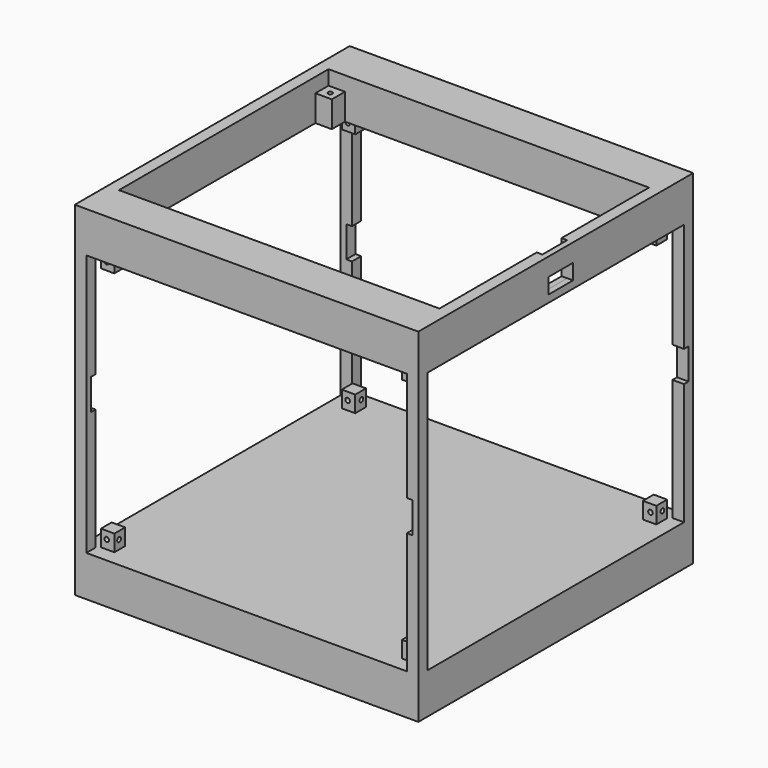
from build123d import *

# Parameters (mm, degrees)
F0_W      = 114.3
F0_H      = 114.3
F1_DEPTH  = 114.3
F2_W      = 5.08
F2_H      = 5.08
F2_R      = 0.762
F2_W_2    = 0.396875
F2_H_2    = 76.2
F3_DEPTH  = 4.826
F2_W_3    = 95.6818
F2_H_3    = 0.396875
F2_H_4    = 30.908625
F2_H_5    = 9.525
F2_H_6    = 34.972625
F4_DEPTH  = 25.4
F2_W_4    = 1.482725
F6_DEPTH  = 11.166475
F5_W      = 10.31875
F5_H      = 5.16255
F7_DEPTH  = 25.4
F11_W     = 5.08
F11_H     = 5.08
F11_R     = 0.762
F12_DEPTH = 4.826
F11_W_2   = 95.6818
F11_H_2   = 0.396875
F11_W_3   = 0.396875
F11_H_3   = 30.908625
F11_H_4   = 34.972625
F11_H_5   = 9.525
F11_H_6   = 76.2
F13_DEPTH = 76.2
F10_W     = 5.08
F10_H     = 5.08
F10_R     = 0.762
F14_DEPTH = 4.826
F10_W_2   = 95.6818
F10_H_2   = 0.396875
F10_W_3   = 0.396875
F10_H_3   = 76.2
F10_H_4   = 34.972625
F10_H_5   = 9.525
F10_H_6   = 30.908625
F15_DEPTH = 50.8
F9_W      = 5.08
F9_H      = 5.08
F9_R      = 0.762
F16_DEPTH = 4.826
F9_W_2    = 95.6818
F9_H_2    = 0.396875
F9_W_3    = 0.396875
F9_H_3    = 76.2
F9_H_4    = 34.972625
F9_H_5    = 9.525
F9_H_6    = 30.908625
F17_DEPTH = 50.8
F8_W      = 5.08
F8_H      = 5.08
F8_R      = 0.762
F18_DEPTH = 4.826
F8_W_2    = 0.396875
F8_H_2    = 76.2
F8_W_3    = 95.6818
F8_H_3    = 0.396875
F8_H_4    = 34.972625
F8_H_5    = 9.525
F8_H_6    = 30.908625
F19_DEPTH = 50.8
F10_W_4   = 1.482725
F20_DEPTH = 11.176
F9_W_4    = 1.482725
F21_DEPTH = 11.176
F8_W_4    = 1.482725
F22_DEPTH = 11.176
F11_W_4   = 1.482725
F23_DEPTH = 11.176


# Not quite as in the source:
# - a feature names something its author has since deleted; it is built from what else it names


with BuildPart() as f1:
    # F0 (on Top) → F1 (new body)
    with BuildSketch(Plane.XY):
        Rectangle(F0_W, F0_H)
    extrude(amount=F1_DEPTH)

    # F2 (on face) → F3 (cut)
    with BuildSketch(Plane.XY.offset(114.3)):
        Polygon((-52.9209, 38.1), (-52.9209, 43.18), (-47.8409, 43.18), (-47.8409, 43.576875), (-53.317775, 43.576875), (-53.317775, 38.1), align=None)
        with Locations((-50.3809, 40.64)):
            Rectangle(F2_W, F2_H)
        with Locations((-50.3809, 40.64)):
            Circle(F2_R, mode=Mode.SUBTRACT)
        with Locations((-53.1193375, 0)):
            Rectangle(F2_W_2, F2_H_2)
        Polygon((47.8409, 43.576875), (47.8409, 43.18), (52.9209, 43.18), (52.9209, 38.1), (53.317775, 38.1), (53.317775, 43.576875), align=None)
        with Locations((50.3809, 40.64)):
            Rectangle(F2_W, F2_H)
        with Locations((50.3809, 40.64)):
            Circle(F2_R, mode=Mode.SUBTRACT)
        with Locations((-50.3809, -40.64)):
            Rectangle(F2_W, F2_H)
        with Locations((-50.3809, -40.64)):
            Circle(F2_R, mode=Mode.SUBTRACT)
        Polygon((-52.9209, -43.18), (-52.9209, -38.1), (-53.317775, -38.1), (-53.317775, -43.576875), (-47.8409, -43.576875), (-47.8409, -43.18), align=None)
        with Locations((50.3809, -40.64)):
            Rectangle(F2_W, F2_H)
        with Locations((50.3809, -40.64)):
            Circle(F2_R, mode=Mode.SUBTRACT)
        Polygon((52.9209, -43.18), (47.8409, -43.18), (47.8409, -43.576875), (53.317775, -43.576875), (53.317775, -38.1), (52.9209, -38.1), align=None)
    extrude(amount=-F3_DEPTH, mode=Mode.SUBTRACT)

    # F2 (on face) → F4 (cut)
    with BuildSketch(Plane.XY.offset(114.3)):
        with Locations((0, 43.3784375)):
            Rectangle(F2_W_3, F2_H_3)
        Polygon((47.8409, 43.18), (-47.8409, 43.18), (-47.8409, 38.1), (-52.9209, 38.1), (-52.9209, -38.1), (-47.8409, -38.1), (-47.8409, -43.18), (47.8409, -43.18), (47.8409, -38.1), (52.9209, -38.1), (52.9209, -3.127375), (52.9209, -2.7305), (52.9209, 6.7945), (52.9209, 7.191375), (52.9209, 38.1), (47.8409, 38.1), align=None)
        with Locations((-53.1193375, 0)):
            Rectangle(F2_W_2, F2_H_2)
        with Locations((53.1193375, 22.6456875)):
            Rectangle(F2_W_2, F2_H_4)
        with Locations((0, -43.3784375)):
            Rectangle(F2_W_3, F2_H_3)
        with Locations((53.1193375, 6.9929375)):
            Rectangle(F2_W_2, F2_H_3)
        with Locations((53.1193375, 2.032)):
            Rectangle(F2_W_2, F2_H_5)
        with Locations((53.1193375, -2.9289375)):
            Rectangle(F2_W_2, F2_H_3)
        with Locations((53.1193375, -20.6136875)):
            Rectangle(F2_W_2, F2_H_6)
        with Locations((-50.3809, -40.64)):
            Circle(F2_R)
        with Locations((50.3809, -40.64)):
            Circle(F2_R)
        with Locations((-50.3809, 40.64)):
            Circle(F2_R)
        with Locations((50.3809, 40.64)):
            Circle(F2_R)
    extrude(amount=-F4_DEPTH, mode=Mode.SUBTRACT)

    # F2 (on face) → F6 (cut)
    with BuildSketch(Plane.XY.offset(114.3)):
        with Locations((-53.1193375, 0)):
            Rectangle(F2_W_2, F2_H_2)
        Polygon((55.197375, 7.191375), (53.317775, 7.191375), (53.317775, 6.7945), (54.8005, 6.7945), (54.8005, -2.7305), (53.317775, -2.7305), (53.317775, -3.127375), (55.197375, -3.127375), align=None)
        with Locations((54.0591375, 2.032)):
            Rectangle(F2_W_4, F2_H_5)
    extrude(amount=-F6_DEPTH, mode=Mode.SUBTRACT)

    # F5 (on face) → F7 (cut)
    with BuildSketch(Plane.YZ.offset(57.15)):
        with Locations((2.032, 105.7402)):
            Rectangle(F5_W, F5_H)
    extrude(amount=-F7_DEPTH, mode=Mode.SUBTRACT)

    # F11 (on face) → F12 (cut)
    with BuildSketch(Plane(origin=(-57.15, 0, 0), x_dir=(0, -1, 0), z_dir=(-1, 0, 0))):
        with Locations((-50.3809, 97.79)):
            Rectangle(F11_W, F11_H)
        with Locations((-50.3809, 97.79)):
            Circle(F11_R, mode=Mode.SUBTRACT)
        Polygon((-52.9209, 95.25), (-52.9209, 100.33), (-47.8409, 100.33), (-47.8409, 100.726875), (-53.317775, 100.726875), (-53.317775, 95.25), align=None)
        Polygon((47.8409, 100.726875), (47.8409, 100.33), (52.9209, 100.33), (52.9209, 95.25), (53.317775, 95.25), (53.317775, 100.726875), align=None)
        with Locations((50.3809, 97.79)):
            Rectangle(F11_W, F11_H)
        with Locations((50.3809, 97.79)):
            Circle(F11_R, mode=Mode.SUBTRACT)
        with Locations((50.3809, 16.51)):
            Rectangle(F11_W, F11_H)
        with Locations((50.3809, 16.51)):
            Circle(F11_R, mode=Mode.SUBTRACT)
        Polygon((52.9209, 13.97), (47.8409, 13.97), (47.8409, 13.573125), (53.317775, 13.573125), (53.317775, 19.05), (52.9209, 19.05), align=None)
        with Locations((-50.3809, 16.51)):
            Rectangle(F11_W, F11_H)
        with Locations((-50.3809, 16.51)):
            Circle(F11_R, mode=Mode.SUBTRACT)
        Polygon((-52.9209, 13.97), (-52.9209, 19.05), (-53.317775, 19.05), (-53.317775, 13.573125), (-47.8409, 13.573125), (-47.8409, 13.97), align=None)
    extrude(amount=-F12_DEPTH, mode=Mode.SUBTRACT)

    # F11 (on face) → F13 (cut)
    with BuildSketch(Plane(origin=(-57.15, 0, 0), x_dir=(0, -1, 0), z_dir=(-1, 0, 0))):
        Polygon((47.8409, 100.33), (-47.8409, 100.33), (-47.8409, 95.25), (-52.9209, 95.25), (-52.9209, 19.05), (-47.8409, 19.05), (-47.8409, 13.97), (47.8409, 13.97), (47.8409, 19.05), (52.9209, 19.05), (52.9209, 54.022625), (52.9209, 54.4195), (52.9209, 63.9445), (52.9209, 64.341375), (52.9209, 95.25), (47.8409, 95.25), align=None)
        with Locations((50.3809, 97.79)):
            Circle(F11_R)
        with Locations((0, 100.5284375)):
            Rectangle(F11_W_2, F11_H_2)
        with Locations((53.1193375, 79.7956875)):
            Rectangle(F11_W_3, F11_H_3)
        with Locations((53.1193375, 36.5363125)):
            Rectangle(F11_W_3, F11_H_4)
        with Locations((50.3809, 16.51)):
            Circle(F11_R)
        with Locations((0, 13.7715625)):
            Rectangle(F11_W_2, F11_H_2)
        with Locations((53.1193375, 54.2210625)):
            Rectangle(F11_W_3, F11_H_2)
        with Locations((53.1193375, 59.182)):
            Rectangle(F11_W_3, F11_H_5)
        with Locations((53.1193375, 64.1429375)):
            Rectangle(F11_W_3, F11_H_2)
        with Locations((-50.3809, 16.51)):
            Circle(F11_R)
        with Locations((-53.1193375, 57.15)):
            Rectangle(F11_W_3, F11_H_6)
        with Locations((-50.3809, 97.79)):
            Circle(F11_R)
    extrude(amount=-F13_DEPTH, mode=Mode.SUBTRACT)

    # F10 (on face) → F14 (cut)
    with BuildSketch(Plane(origin=(0, 57.15, 0), x_dir=(-1, 0, 0), z_dir=(0, 1, 0))):
        Polygon((-52.9209, 95.25), (-52.9209, 100.33), (-47.8409, 100.33), (-47.8409, 100.726875), (-53.317775, 100.726875), (-53.317775, 95.25), align=None)
        with Locations((-50.3809, 97.79)):
            Rectangle(F10_W, F10_H)
        with Locations((-50.3809, 97.79)):
            Circle(F10_R, mode=Mode.SUBTRACT)
        Polygon((47.8409, 100.726875), (47.8409, 100.33), (52.9209, 100.33), (52.9209, 95.25), (53.317775, 95.25), (53.317775, 100.726875), align=None)
        with Locations((50.3809, 97.79)):
            Rectangle(F10_W, F10_H)
        with Locations((50.3809, 97.79)):
            Circle(F10_R, mode=Mode.SUBTRACT)
        with Locations((50.3809, 16.51)):
            Rectangle(F10_W, F10_H)
        with Locations((50.3809, 16.51)):
            Circle(F10_R, mode=Mode.SUBTRACT)
        Polygon((52.9209, 13.97), (47.8409, 13.97), (47.8409, 13.573125), (53.317775, 13.573125), (53.317775, 19.05), (52.9209, 19.05), align=None)
        Polygon((-52.9209, 13.97), (-52.9209, 19.05), (-53.317775, 19.05), (-53.317775, 13.573125), (-47.8409, 13.573125), (-47.8409, 13.97), align=None)
        with Locations((-50.3809, 16.51)):
            Rectangle(F10_W, F10_H)
        with Locations((-50.3809, 16.51)):
            Circle(F10_R, mode=Mode.SUBTRACT)
    extrude(amount=-F14_DEPTH, mode=Mode.SUBTRACT)

    # F10 (on face) → F15 (cut)
    with BuildSketch(Plane(origin=(0, 57.15, 0), x_dir=(-1, 0, 0), z_dir=(0, 1, 0))):
        Polygon((47.8409, 100.33), (-47.8409, 100.33), (-47.8409, 95.25), (-52.9209, 95.25), (-52.9209, 19.05), (-47.8409, 19.05), (-47.8409, 13.97), (47.8409, 13.97), (47.8409, 19.05), (52.9209, 19.05), (52.9209, 54.022625), (52.9209, 54.4195), (52.9209, 63.9445), (52.9209, 64.341375), (52.9209, 95.25), (47.8409, 95.25), align=None)
        with Locations((0, 100.5284375)):
            Rectangle(F10_W_2, F10_H_2)
        with Locations((-53.1193375, 57.15)):
            Rectangle(F10_W_3, F10_H_3)
        with Locations((0, 13.7715625)):
            Rectangle(F10_W_2, F10_H_2)
        with Locations((53.1193375, 36.5363125)):
            Rectangle(F10_W_3, F10_H_4)
        with Locations((53.1193375, 54.2210625)):
            Rectangle(F10_W_3, F10_H_2)
        with Locations((53.1193375, 59.182)):
            Rectangle(F10_W_3, F10_H_5)
        with Locations((53.1193375, 64.1429375)):
            Rectangle(F10_W_3, F10_H_2)
        with Locations((53.1193375, 79.7956875)):
            Rectangle(F10_W_3, F10_H_6)
        with Locations((-50.3809, 97.79)):
            Circle(F10_R)
        with Locations((50.3809, 97.79)):
            Circle(F10_R)
        with Locations((50.3809, 16.51)):
            Circle(F10_R)
        with Locations((-50.3809, 16.51)):
            Circle(F10_R)
    extrude(amount=-F15_DEPTH, mode=Mode.SUBTRACT)

    # F9 (on face) → F16 (cut)
    with BuildSketch(Plane.YZ.offset(57.15)):
        Polygon((-52.9209, 95.25), (-52.9209, 100.33), (-47.8409, 100.33), (-47.8409, 100.726875), (-53.317775, 100.726875), (-53.317775, 95.25), align=None)
        with Locations((-50.3809, 97.79)):
            Rectangle(F9_W, F9_H)
        with Locations((-50.3809, 97.79)):
            Circle(F9_R, mode=Mode.SUBTRACT)
        Polygon((47.8409, 100.726875), (47.8409, 100.33), (52.9209, 100.33), (52.9209, 95.25), (53.317775, 95.25), (53.317775, 100.726875), align=None)
        with Locations((50.3809, 97.79)):
            Rectangle(F9_W, F9_H)
        with Locations((50.3809, 97.79)):
            Circle(F9_R, mode=Mode.SUBTRACT)
        Polygon((52.9209, 13.97), (47.8409, 13.97), (47.8409, 13.573125), (53.317775, 13.573125), (53.317775, 19.05), (52.9209, 19.05), align=None)
        with Locations((50.3809, 16.51)):
            Rectangle(F9_W, F9_H)
        with Locations((50.3809, 16.51)):
            Circle(F9_R, mode=Mode.SUBTRACT)
        Polygon((-52.9209, 13.97), (-52.9209, 19.05), (-53.317775, 19.05), (-53.317775, 13.573125), (-47.8409, 13.573125), (-47.8409, 13.97), align=None)
        with Locations((-50.3809, 16.51)):
            Rectangle(F9_W, F9_H)
        with Locations((-50.3809, 16.51)):
            Circle(F9_R, mode=Mode.SUBTRACT)
    extrude(amount=-F16_DEPTH, mode=Mode.SUBTRACT)

    # F9 (on face) → F17 (cut)
    with BuildSketch(Plane.YZ.offset(57.15)):
        Polygon((47.8409, 100.33), (-47.8409, 100.33), (-47.8409, 95.25), (-52.9209, 95.25), (-52.9209, 19.05), (-47.8409, 19.05), (-47.8409, 13.97), (47.8409, 13.97), (47.8409, 19.05), (52.9209, 19.05), (52.9209, 54.022625), (52.9209, 54.4195), (52.9209, 63.9445), (52.9209, 64.341375), (52.9209, 95.25), (47.8409, 95.25), align=None)
        with Locations((0, 13.7715625)):
            Rectangle(F9_W_2, F9_H_2)
        with Locations((-53.1193375, 57.15)):
            Rectangle(F9_W_3, F9_H_3)
        with Locations((53.1193375, 36.5363125)):
            Rectangle(F9_W_3, F9_H_4)
        with Locations((53.1193375, 54.2210625)):
            Rectangle(F9_W_3, F9_H_2)
        with Locations((53.1193375, 59.182)):
            Rectangle(F9_W_3, F9_H_5)
        with Locations((53.1193375, 64.1429375)):
            Rectangle(F9_W_3, F9_H_2)
        with Locations((53.1193375, 79.7956875)):
            Rectangle(F9_W_3, F9_H_6)
        with Locations((0, 100.5284375)):
            Rectangle(F9_W_2, F9_H_2)
        with Locations((50.3809, 16.51)):
            Circle(F9_R)
        with Locations((50.3809, 97.79)):
            Circle(F9_R)
        with Locations((-50.3809, 97.79)):
            Circle(F9_R)
        with Locations((-50.3809, 16.51)):
            Circle(F9_R)
    extrude(amount=-F17_DEPTH, mode=Mode.SUBTRACT)

    # F8 (on face) → F18 (cut)
    with BuildSketch(Plane.XZ.offset(57.15)):
        with Locations((-50.3809, 97.79)):
            Rectangle(F8_W, F8_H)
        with Locations((-50.3809, 97.79)):
            Circle(F8_R, mode=Mode.SUBTRACT)
        Polygon((-52.9209, 95.25), (-52.9209, 100.33), (-47.8409, 100.33), (-47.8409, 100.726875), (-53.317775, 100.726875), (-53.317775, 95.25), align=None)
        Polygon((47.8409, 100.726875), (47.8409, 100.33), (52.9209, 100.33), (52.9209, 95.25), (53.317775, 95.25), (53.317775, 100.726875), align=None)
        with Locations((50.3809, 97.79)):
            Rectangle(F8_W, F8_H)
        with Locations((50.3809, 97.79)):
            Circle(F8_R, mode=Mode.SUBTRACT)
        Polygon((52.9209, 13.97), (47.8409, 13.97), (47.8409, 13.573125), (53.317775, 13.573125), (53.317775, 19.05), (52.9209, 19.05), align=None)
        with Locations((50.3809, 16.51)):
            Rectangle(F8_W, F8_H)
        with Locations((50.3809, 16.51)):
            Circle(F8_R, mode=Mode.SUBTRACT)
        Polygon((-52.9209, 13.97), (-52.9209, 19.05), (-53.317775, 19.05), (-53.317775, 13.573125), (-47.8409, 13.573125), (-47.8409, 13.97), align=None)
        with Locations((-50.3809, 16.51)):
            Rectangle(F8_W, F8_H)
        with Locations((-50.3809, 16.51)):
            Circle(F8_R, mode=Mode.SUBTRACT)
    extrude(amount=-F18_DEPTH, mode=Mode.SUBTRACT)

    # F8 (on face) → F19 (cut)
    with BuildSketch(Plane.XZ.offset(57.15)):
        Polygon((47.8409, 100.33), (-47.8409, 100.33), (-47.8409, 95.25), (-52.9209, 95.25), (-52.9209, 19.05), (-47.8409, 19.05), (-47.8409, 13.97), (47.8409, 13.97), (47.8409, 19.05), (52.9209, 19.05), (52.9209, 54.022625), (52.9209, 54.4195), (52.9209, 63.9445), (52.9209, 64.341375), (52.9209, 95.25), (47.8409, 95.25), align=None)
        with Locations((-50.3809, 16.51)):
            Circle(F8_R)
        with Locations((-53.1193375, 57.15)):
            Rectangle(F8_W_2, F8_H_2)
        with Locations((0, 13.7715625)):
            Rectangle(F8_W_3, F8_H_3)
        with Locations((53.1193375, 36.5363125)):
            Rectangle(F8_W_2, F8_H_4)
        with Locations((50.3809, 16.51)):
            Circle(F8_R)
        with Locations((53.1193375, 54.2210625)):
            Rectangle(F8_W_2, F8_H_3)
        with Locations((53.1193375, 59.182)):
            Rectangle(F8_W_2, F8_H_5)
        with Locations((53.1193375, 64.1429375)):
            Rectangle(F8_W_2, F8_H_3)
        with Locations((53.1193375, 79.7956875)):
            Rectangle(F8_W_2, F8_H_6)
        with Locations((0, 100.5284375)):
            Rectangle(F8_W_3, F8_H_3)
        with Locations((-50.3809, 97.79)):
            Circle(F8_R)
        with Locations((50.3809, 97.79)):
            Circle(F8_R)
    extrude(amount=-F19_DEPTH, mode=Mode.SUBTRACT)

    # F10 (on face) → F20 (cut)
    with BuildSketch(Plane(origin=(0, 57.15, 0), x_dir=(-1, 0, 0), z_dir=(0, 1, 0))):
        Polygon((55.197375, 64.341375), (53.317775, 64.341375), (53.317775, 63.9445), (54.8005, 63.9445), (54.8005, 54.4195), (53.317775, 54.4195), (53.317775, 54.022625), (55.197375, 54.022625), align=None)
        with Locations((54.0591375, 59.182)):
            Rectangle(F10_W_4, F10_H_5)
    extrude(amount=-F20_DEPTH, mode=Mode.SUBTRACT)

    # F9 (on face) → F21 (cut)
    with BuildSketch(Plane.YZ.offset(57.15)):
        with Locations((54.0591375, 59.182)):
            Rectangle(F9_W_4, F9_H_5)
        Polygon((55.197375, 64.341375), (53.317775, 64.341375), (53.317775, 63.9445), (54.8005, 63.9445), (54.8005, 54.4195), (53.317775, 54.4195), (53.317775, 54.022625), (55.197375, 54.022625), align=None)
    extrude(amount=-F21_DEPTH, mode=Mode.SUBTRACT)

    # F8 (on face) → F22 (cut)
    with BuildSketch(Plane.XZ.offset(57.15)):
        with Locations((54.0591375, 59.182)):
            Rectangle(F8_W_4, F8_H_5)
        Polygon((55.197375, 64.341375), (53.317775, 64.341375), (53.317775, 63.9445), (54.8005, 63.9445), (54.8005, 54.4195), (53.317775, 54.4195), (53.317775, 54.022625), (55.197375, 54.022625), align=None)
    extrude(amount=-F22_DEPTH, mode=Mode.SUBTRACT)

    # F11 (on face) → F23 (cut)
    with BuildSketch(Plane(origin=(-57.15, 0, 0), x_dir=(0, -1, 0), z_dir=(-1, 0, 0))):
        Polygon((55.197375, 64.341375), (53.317775, 64.341375), (53.317775, 63.9445), (54.8005, 63.9445), (54.8005, 54.4195), (53.317775, 54.4195), (53.317775, 54.022625), (55.197375, 54.022625), align=None)
        with Locations((54.0591375, 59.182)):
            Rectangle(F11_W_4, F11_H_5)
    extrude(amount=-F23_DEPTH, mode=Mode.SUBTRACT)


solid = f1.part
